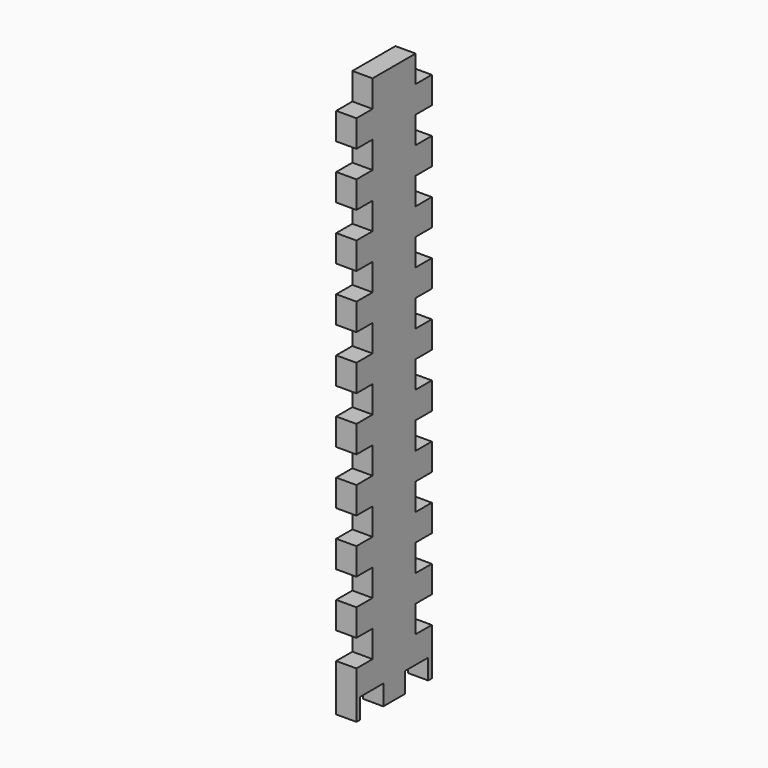
from build123d import *

# Parameters (mm, degrees)
F0_W     = 24
F0_H     = 240
F1_DEPTH = 9
F2_W     = 9
F2_H     = 12
F3_DEPTH = 9
F4_W     = 12
F4_H     = 9
F4_W_2   = 2
F5_DEPTH = 9


with BuildPart() as f1:
    # F0 (on Right) → F1 (new body)
    with BuildSketch(Plane.YZ):
        Rectangle(F0_W, F0_H)
    extrude(amount=F1_DEPTH)

    # F2 (on face) → F3 (join, through all)
    with BuildSketch(Plane.YZ.offset(9)):
        with Locations((-16.5, -114)):
            Rectangle(F2_W, F2_H)
        with Locations((-16.5, -90)):
            Rectangle(F2_W, F2_H)
        with Locations((-16.5, -66)):
            Rectangle(F2_W, F2_H)
        with Locations((-16.5, -42)):
            Rectangle(F2_W, F2_H)
        with Locations((-16.5, -18)):
            Rectangle(F2_W, F2_H)
        with Locations((-16.5, 6)):
            Rectangle(F2_W, F2_H)
        with Locations((-16.5, 30)):
            Rectangle(F2_W, F2_H)
        with Locations((-16.5, 54)):
            Rectangle(F2_W, F2_H)
        with Locations((-16.5, 78)):
            Rectangle(F2_W, F2_H)
        with Locations((-16.5, 102)):
            Rectangle(F2_W, F2_H)
        with Locations((16.5, -90)):
            Rectangle(F2_W, F2_H)
        with Locations((16.5, 30)):
            Rectangle(F2_W, F2_H)
        with Locations((16.5, 102)):
            Rectangle(F2_W, F2_H)
        with Locations((16.5, -18)):
            Rectangle(F2_W, F2_H)
        with Locations((16.5, 78)):
            Rectangle(F2_W, F2_H)
        with Locations((16.5, 6)):
            Rectangle(F2_W, F2_H)
        with Locations((16.5, 54)):
            Rectangle(F2_W, F2_H)
        with Locations((16.5, -42)):
            Rectangle(F2_W, F2_H)
        with Locations((16.5, -66)):
            Rectangle(F2_W, F2_H)
        with Locations((16.5, -114)):
            Rectangle(F2_W, F2_H)
    extrude(amount=-F3_DEPTH)

    # F4 (on face) → F5 (join, through all)
    with BuildSketch(Plane.YZ.offset(9)):
        with Locations((0, -124.5)):
            Rectangle(F4_W, F4_H)
        with Locations((20, -124.5)):
            Rectangle(F4_W_2, F4_H)
        with Locations((-20, -124.5)):
            Rectangle(F4_W_2, F4_H)
    extrude(amount=-F5_DEPTH)


solid = f1.part
